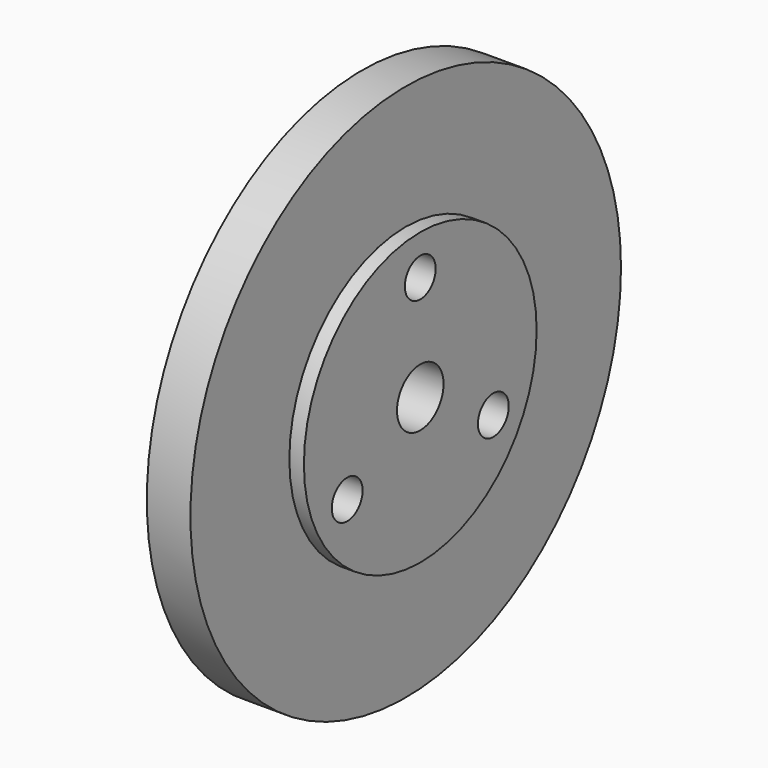
from build123d import *

# Parameters (mm, degrees)
F0_R     = 37
F0_R_2   = 20
F0_R_3   = 2.65
F0_R_4   = 4
F1_DEPTH = 8
F2_DEPTH = 2


# Not quite as in the source:
# - a feature names something its author has since deleted; it is built from what else it names


with BuildPart() as f1:
    # F0 (on Right) → F1 (new body)
    with BuildSketch(Plane.YZ):
        Circle(F0_R)
        Circle(F0_R_2, mode=Mode.SUBTRACT)
        Circle(F0_R_2)
        with Locations((-12.5573683549, -7.25)):
            Circle(F0_R_3, mode=Mode.SUBTRACT)
        with Locations((12.5573683549, -7.25)):
            Circle(F0_R_3, mode=Mode.SUBTRACT)
        Circle(F0_R_4, mode=Mode.SUBTRACT)
        with Locations((0, 14.5)):
            Circle(F0_R_3, mode=Mode.SUBTRACT)
    extrude(amount=-F1_DEPTH)

    # F0 (on Right) → F2 (cut)
    with BuildSketch(Plane.YZ):
        Circle(F0_R)
        Circle(F0_R_2, mode=Mode.SUBTRACT)
    extrude(amount=-F2_DEPTH, mode=Mode.SUBTRACT)


solid = f1.part
